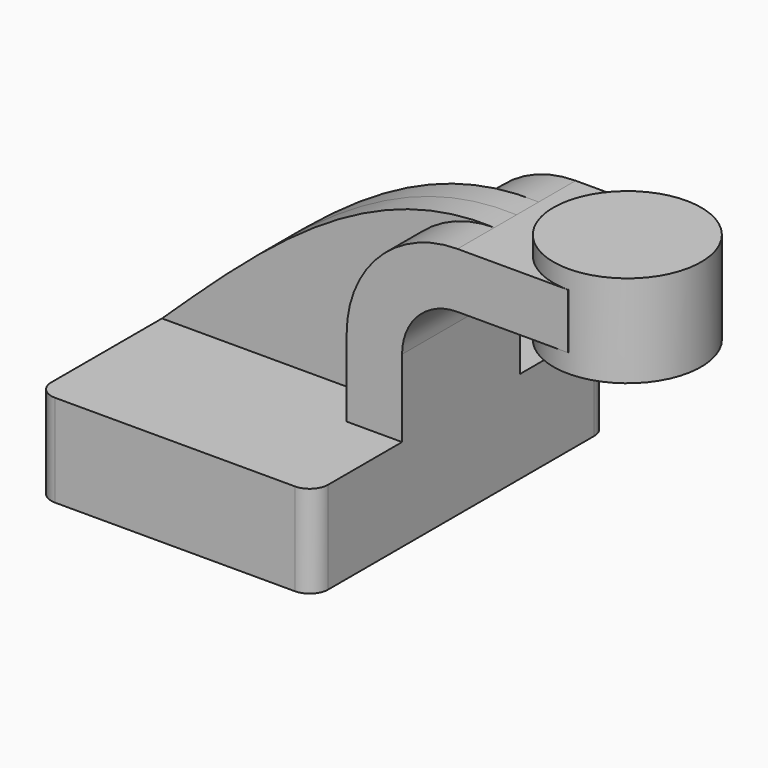
from build123d import *

# Parameters (mm, degrees)
F0_W          = 20.32
F0_H          = 15.24000009
F0_H_2        = 5.07999991
F0_H_3        = 5.08
F2_DEPTH      = 50.8
F2_DEPTH_BACK = 50.8
F3_DEPTH      = 20.32
F3_DEPTH_BACK = 20.32
F4_DEPTH      = 7.62
F4_DEPTH_BACK = 7.62
F5_R          = 5.08


with BuildPart() as f1:
    # F0 (on Front) → F1 (revolve)
    with BuildSketch(Plane.XZ):
        with Locations((73.66, 56.8193151802)):
            Rectangle(F0_W, F0_H)
        with Locations((73.66, 66.9793151802)):
            Rectangle(F0_W, F0_H_2)
        with Locations((73.66, 46.6593151352)):
            Rectangle(F0_W, F0_H_3)
    revolve(axis=Axis((83.82, 0, 63.1609670818), (0, 0, -1)))


with BuildPart() as f2:
    # F0 (on Front) → F2 (new body, two sides)
    with BuildSketch(Plane.XZ) as f2_sk:
        Polygon((-38.1, -12.7), (38.1, -12.7), (38.1, 12.7), (22.85999991, 12.7), (-38.1, 12.7), align=None)
    extrude(amount=F2_DEPTH)
    extrude(f2_sk.sketch, amount=-F2_DEPTH_BACK)

    # F0 (on Front) → F3 (join, two sides)
    with BuildSketch(Plane.XZ) as f3_sk:
        with Locations((73.66, 56.8193151802)):
            Rectangle(F0_W, F0_H)
        with BuildLine():
            Line((22.85999991, 12.7), (38.1, 12.7))
            Line((38.1, 12.7), (38.1, 33.9593151352))
            ThreePointArc((38.1, 33.9593151352), (42.5636926547, 44.7356224805), (53.34, 49.1993151352))
            Line((53.34, 49.1993151352), (63.5, 49.1993151352))
            Line((63.5, 49.1993151352), (63.5, 64.4393152252))
            Line((63.5, 64.4393152252), (53.34, 64.4393152252))
            ThreePointArc((53.34, 64.4393152252), (31.7873852458, 55.5119298894), (22.85999991, 33.9593151352))
            Line((22.85999991, 33.9593151352), (22.85999991, 12.7))
        make_face()
    extrude(amount=F3_DEPTH)
    extrude(f3_sk.sketch, amount=-F3_DEPTH_BACK)

    # F0 (on Front) → F4 (join, two sides)
    with BuildSketch(Plane.XZ) as f4_sk:
        with BuildLine():
            add(Edge.make_bspline(
                [(53.34, 64.4393152252), (18.0031490481, 65.8844992586), (-10.2887663049, 39.0674972777), (-38.1, 12.7)],
                knots=[0, 0, 0, 0, 105.0629827293, 105.0629827293, 105.0629827293, 105.0629827293], degree=3))
            Line((-38.1, 12.7), (22.85999991, 12.7))
            Line((22.85999991, 12.7), (22.85999991, 33.9593151352))
            ThreePointArc((22.85999991, 33.9593151352), (31.7873852458, 55.5119298894), (53.34, 64.4393152252))
        make_face()
    extrude(amount=F4_DEPTH)
    extrude(f4_sk.sketch, amount=-F4_DEPTH_BACK)

    # F5
    f5_edges = [f2.edges().sort_by_distance(p)[0] for p in [
        (-38.1, -50.8, 0),
        (38.1, -50.8, 0),
        (-38.1, 50.8, 0),
        (38.1, 50.8, 0),
    ]]
    fillet(f5_edges, radius=F5_R)


solid = Compound([f1.part, f2.part])
